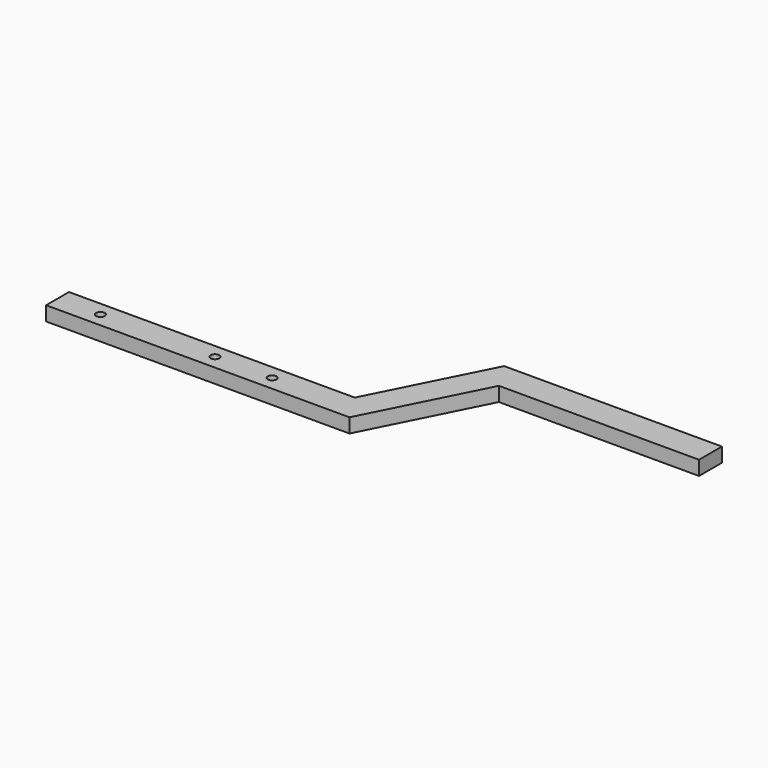
from build123d import *

# Parameters (mm, degrees)
F0_R     = 1.5
F1_DEPTH = 5
F2_DEPTH = 265


# Not quite as in the source:
# - an extrude ends at something that could not be found from the text; its depth is read off the source's solid


with BuildPart() as f1:
    # F0 (on Top) → F1 (new body)
    with BuildSketch(Plane.XY):
        Polygon((-52.0408339798, -45.9276453106), (-151.9144345724, -45.9276453106), (-151.9144345724, -55.9276454151), (-45.8887560524, -55.9276454151), (-25.683571109, -15.9276453106), (27.9570557177, -15.9276453106), (44.264588505, -15.9276453106), (44.264588505, -5.9276453106), (27.9570557177, -5.9276453106), (-31.8356490892, -5.9276453106), (-31.9144345724, -6.0836161342), align=None)
        with Locations((-136.9144345724, -50.9276454151)):
            Circle(F0_R, mode=Mode.SUBTRACT)
        with Locations((-96.9144345724, -50.9276454151)):
            Circle(F0_R, mode=Mode.SUBTRACT)
        with Locations((-76.9144345724, -50.9276454151)):
            Circle(F0_R, mode=Mode.SUBTRACT)
    extrude(amount=F1_DEPTH)

    # F0 (on Top) → F2 (cut, through all)
    with BuildSketch(Plane.XY):
        with Locations((-76.9144345724, -50.9276454151)):
            Circle(F0_R)
        with Locations((-96.9144345724, -50.9276454151)):
            Circle(F0_R)
    extrude(amount=-F2_DEPTH, mode=Mode.SUBTRACT)


solid = f1.part
